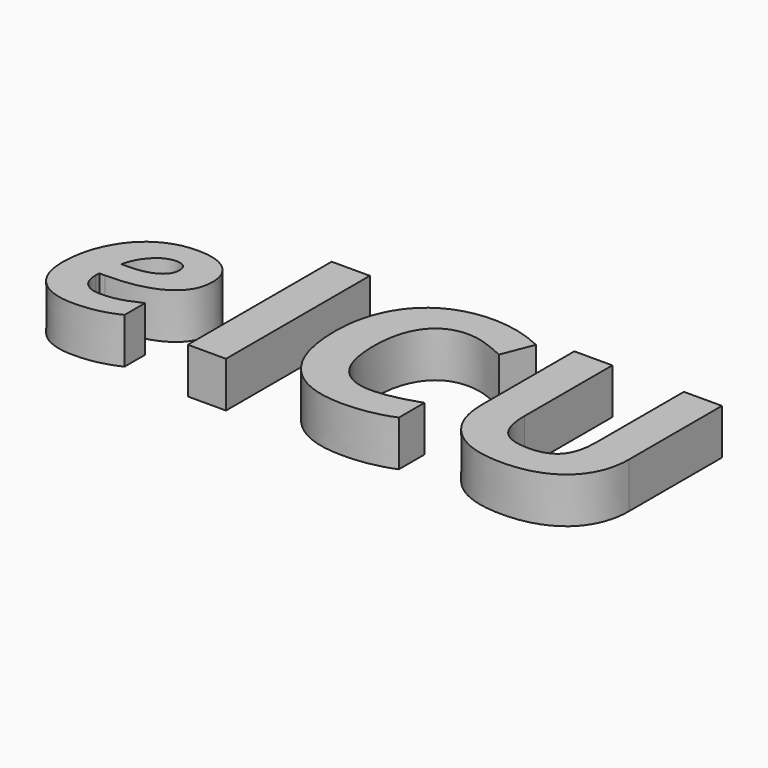
from build123d import *

# Parameters (mm, degrees)
F0_TEXT_SIZE   = 7.0180934535
F0_TEXT_SIZE_2 = 6.4216957109
F1_DEPTH       = 1.27


# Not quite as in the source:
# - Text() gives the source's letters only with a copy of the font that has no kerning and outlines rounded to 1/6400 em; it was checked with that copy


with BuildPart() as f1:
    # F0 (on Top) → F1 (new body)
    with BuildSketch(Plane.XY):
        with Locations((4.2126021043, -0.0313776831)):
            Text('ICU', F0_TEXT_SIZE, font='Open Sans', font_style=FontStyle.BOLD, text_align=(TextAlign.LEFT, TextAlign.BOTTOM))
        with Locations((0, 0)):
            Text('e', F0_TEXT_SIZE_2, font='Open Sans', font_style=FontStyle.BOLDITALIC, text_align=(TextAlign.LEFT, TextAlign.BOTTOM))
    extrude(amount=F1_DEPTH)


solid = f1.part
